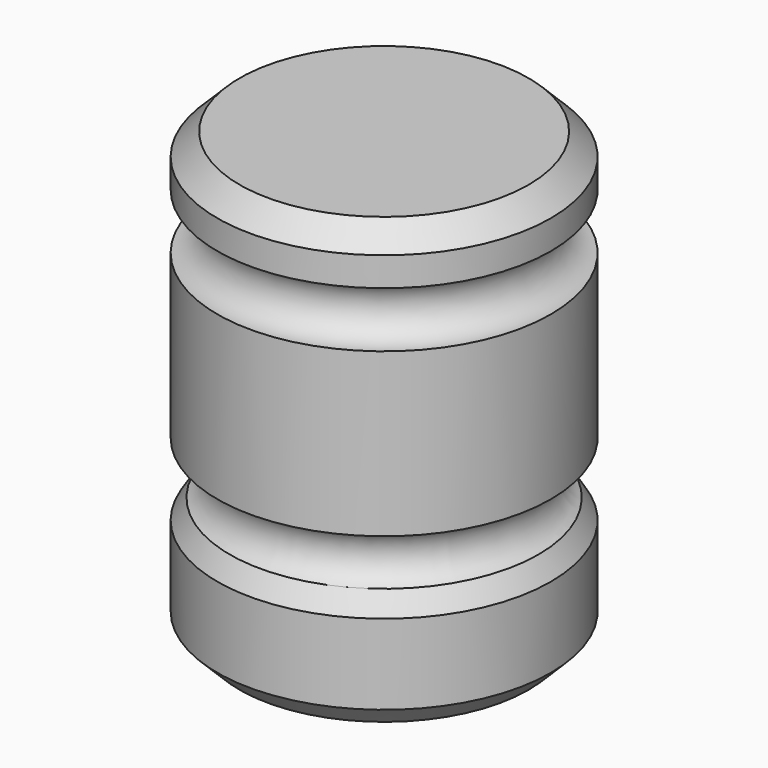
from build123d import *


# Not quite as in the source:
# - a fillet or chamfer that OpenCascade refuses, or shapes differently, is made with other operations: its cross-section is extruded or revolved along the edge and cut away or added


with BuildPart() as f1:
    # F0 (on Front) → F1 (revolve)
    with BuildSketch(Plane.XZ):
        with BuildLine():
            Line((-38.1, 0), (0, 0))
            Line((0, 0), (0, 27.2913607001))
            ThreePointArc((0, 27.2913607001), (-6.35, 33.6413607001), (0, 39.9913607001))
            Line((0, 39.9913607001), (0, 77.1941723466))
            ThreePointArc((0, 77.1941723466), (-6.35, 83.5441723466), (0, 89.8941723466))
            Line((0, 89.8941723466), (0, 101.6))
            Line((0, 101.6), (-38.1, 101.6))
            Line((-38.1, 101.6), (-38.1, 0))
        make_face()
    revolve(axis=Axis((-38.1, 0, 50.8), (0, 0, 1)))

    # F2: chamfer of 5.08 on 4 edges, made by hand

    # F2_s1 → F2_t2 (revolve, cut)
    with BuildSketch(Plane.XZ):
        Polygon((0, 96.52), (-5.08, 101.6), (0, 101.6), align=None)
    revolve(axis=Axis((-38.1, 0, 101.6), (0, 0, 1)), mode=Mode.SUBTRACT)

    # F2_s3 → F2_t4 (revolve, cut)
    with BuildSketch(Plane.XZ):
        Polygon((-5.08, 0), (0, 5.08), (0, 0), align=None)
    revolve(axis=Axis((-38.1, 0, 0), (0, 0, 1)), mode=Mode.SUBTRACT)

    # F2_s5 → F2_t6 (revolve, cut)
    with BuildSketch(Plane.XZ):
        with BuildLine():
            Line((0, 23.4022933598), (-2.8222222222, 27.9529899555))
            ThreePointArc((-2.8222222222, 27.9529899555), (-1.5219513398, 27.4764467413), (0, 27.2913607001))
            Line((0, 27.2913607001), (0, 23.4022933598))
        make_face()
    revolve(axis=Axis((-38.1, 0, 27.2913607001), (0, 0, 1)), mode=Mode.SUBTRACT)


solid = f1.part
